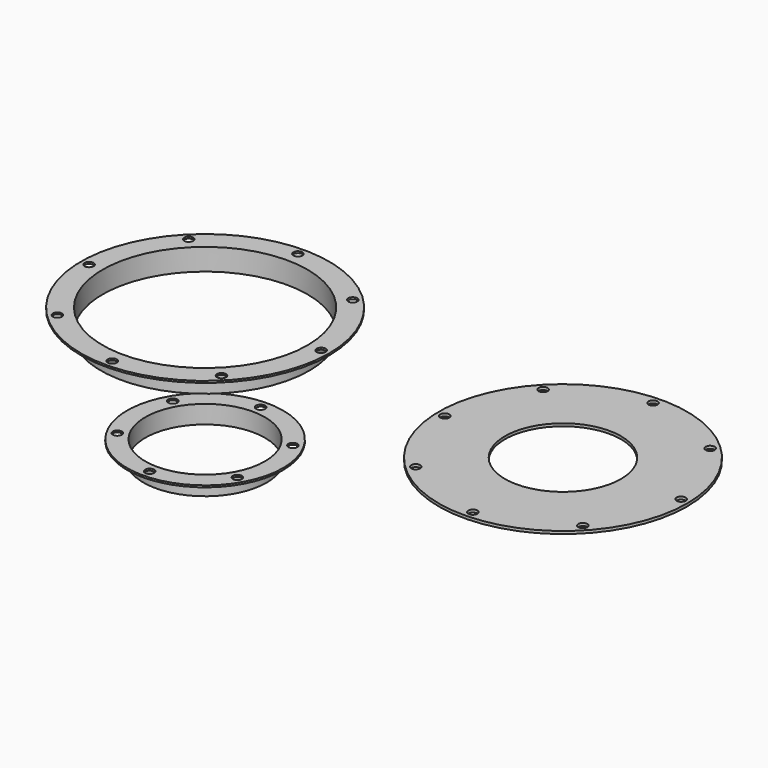
from build123d import *

# Parameters (mm, degrees)
F2_R             = 7.9375
F3_DEPTH         = 25.4
F3_COPIES_COUNT  = 6
F6_R             = 7.9375
F7_DEPTH         = 25.4
F7_COPIES_COUNT  = 8
F8_R             = 217.4875
F9_DEPTH         = 4.7625
F10_R            = 7.9375
F11_DEPTH        = 25.4
F11_COPIES_COUNT = 8
F12_R            = 101.6
F13_DEPTH        = 25.4


# Not quite as in the source:
# - a pattern or mirror of a feature is missing from the dataset's text; its kind, count and spacing are read off the source's solid


with BuildPart() as f1:
    # F0 (on Front) → F1 (revolve)
    with BuildSketch(Plane.XZ):
        Polygon((136.525, 0), (104.775, 0), (104.775, -31.75), (107.95, -31.75), (107.95, -3.175), (136.525, -3.175), align=None)
    revolve(axis=Axis((0, 0, 35.2586749941), (0, 0, -1)))

    # F2 (on face) → F3 (cut)
    with BuildSketch(Plane.XY):
        with Locations((0, 121.44375)):
            Circle(F2_R)
    f3 = extrude(amount=-F3_DEPTH, mode=Mode.SUBTRACT)

    # F3_copies: F3 ×6 about axis
    f3_copies_axis = Axis((0, 0, 0), (0, 0, 1))
    for i in range(1, F3_COPIES_COUNT):
        add(f3.rotate(f3_copies_axis, i * 360 / F3_COPIES_COUNT), mode=Mode.SUBTRACT)


with BuildPart() as f5:
    # F4 (on Front) → F5 (revolve)
    with BuildSketch(Plane.XZ):
        Polygon((217.4875, 203.2), (179.3875, 203.2), (179.3875, 165.1), (182.5625, 165.1), (182.5625, 200.025), (217.4875, 200.025), align=None)
    revolve(axis=Axis((0, 0, 35.2586749941), (0, 0, -1)))

    # F6 (on face) → F7 (cut)
    with BuildSketch(Plane.XY.offset(203.2)):
        with Locations((0, 203.2)):
            Circle(F6_R)
    f7 = extrude(amount=-F7_DEPTH, mode=Mode.SUBTRACT)

    # F7_copies: F7 ×8 about axis
    f7_copies_axis = Axis((0, 0, 0), (0, 0, 1))
    for i in range(1, F7_COPIES_COUNT):
        add(f7.rotate(f7_copies_axis, i * 360 / F7_COPIES_COUNT), mode=Mode.SUBTRACT)


with BuildPart() as f9:
    # F8 (on Top) → F9 (new body)
    with BuildSketch(Plane.XY):
        with Locations((421.7100143433, 256.2264800072)):
            Circle(F8_R)
    extrude(amount=F9_DEPTH)

    # F10 (on face) → F11 (cut)
    with BuildSketch(Plane.XY.offset(4.7625)):
        with Locations((416.9476355011, 459.3706646342)):
            Circle(F10_R)
    f11 = extrude(amount=-F11_DEPTH, mode=Mode.SUBTRACT)

    # F11_copies: F11 ×8 about axis
    f11_copies_axis = Axis((421.710014, 256.22648, 0), (0, 0, 1))
    for i in range(1, F11_COPIES_COUNT):
        add(f11.rotate(f11_copies_axis, i * 360 / F11_COPIES_COUNT), mode=Mode.SUBTRACT)

    # F12 (on face) → F13 (cut)
    with BuildSketch(Plane.XY.offset(4.7625)):
        with Locations((421.7100143433, 256.2264800072)):
            Circle(F12_R)
    extrude(amount=-F13_DEPTH, mode=Mode.SUBTRACT)


solid = Compound([f1.part, f5.part, f9.part])
